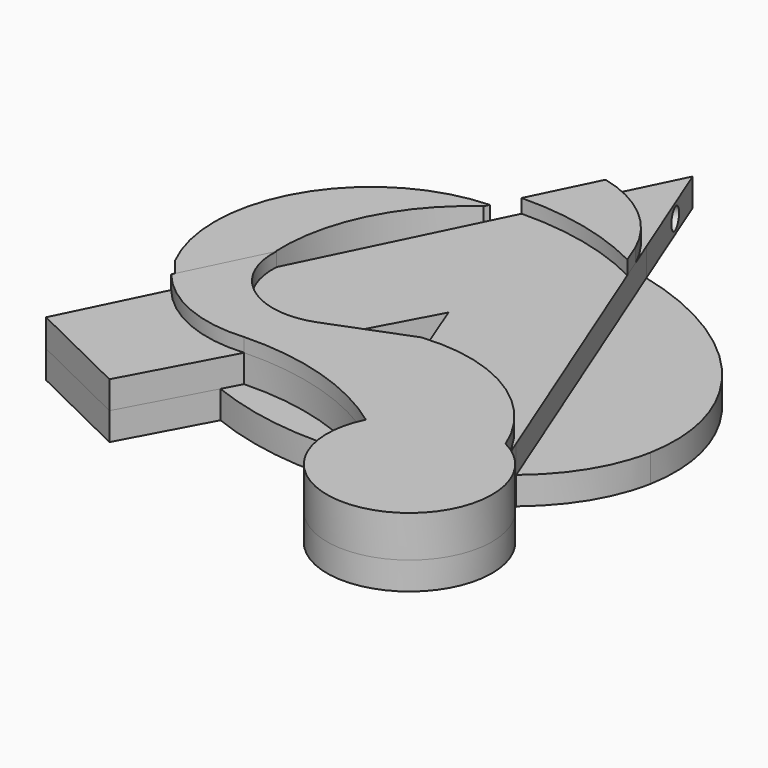
from build123d import *

# Parameters (mm, degrees)
F1_DEPTH  = 5.08
F3_DEPTH  = 5.08
F5_DEPTH  = 2.54
F7_DEPTH  = 10.16
F8_DEPTH  = 5.08
F9_DEPTH  = 5.08
F11_DEPTH = 7.62
F12_DEPTH = 2.54
F13_R     = 1.905


with BuildPart() as f1:
    # F0 (on Top) → F1 (new body)
    with BuildSketch(Plane.XY):
        with BuildLine():
            add(Edge.make_bspline(
                [(-53.1635676672, -40.7425994368), (-41.8989411061, 18.6911877843), (-113.0400156659, 1.3903249669), (-184.1810902258, -15.9105378505), (-124.304642227, -58.0434622542), (-64.4281942283, -100.1763866579), (-53.1635676672, -40.7425994368)],
                knots=[0, 0, 0, 2.0943951024, 2.0943951024, 4.1887902048, 4.1887902048, 6.2831853072, 6.2831853072, 6.2831853072], degree=2, weights=[1, 0.5, 1, 0.5, 1, 0.5, 1]))
        make_face()
    extrude(amount=F1_DEPTH)

    # F2 (on face) → F3 (join)
    with BuildSketch(Plane.XY.offset(5.08)):
        with BuildLine():
            Line((-131.9579197109, -51.2809136758), (-140.9604847431, -69.6664303541))
            Line((-140.9604847431, -69.6664303541), (-121.8411935672, -79.0282919321))
            Line((-121.8411935672, -79.0282919321), (-113.6531802251, -63.7810597846))
            add(Edge.make_bspline(
                [(-131.9579197109, -51.2809136758), (-128.6186368439, -55.0078578531), (-124.304642227, -58.0434622542), (-119.420845427, -61.4800161624), (-113.6531802251, -63.7810597846)],
                knots=[3.9072776048, 3.9072776048, 3.9072776048, 4.1887902048, 4.1887902048, 4.50468154, 4.50468154, 4.50468154], degree=2, weights=[0.8836543185, 0.9327938173, 1, 0.9245864988, 0.8719217822]))
        make_face()
        with BuildLine():
            Line((-105.5654466698, 2.6191971859), (-131.9579197109, -51.2809136758))
            add(Edge.make_bspline(
                [(-131.9579197109, -51.2809136758), (-128.6186368439, -55.0078578531), (-124.304642227, -58.0434622542), (-119.420845427, -61.4800161624), (-113.6531802251, -63.7810597846)],
                knots=[3.9072776048, 3.9072776048, 3.9072776048, 4.1887902048, 4.1887902048, 4.50468154, 4.50468154, 4.50468154], degree=2, weights=[0.8836543185, 0.9327938173, 1, 0.9245864988, 0.8719217822]))
            Line((-113.6531802251, -63.7810597846), (-96.8360751867, -32.4652455747))
            Line((-96.8360751867, -32.4652455747), (-83.3206423237, -66.8956124574))
            add(Edge.make_bspline(
                [(-83.3206423237, -66.8956124574), (-71.8467350955, -64.7720622624), (-63.8384492188, -58.1680738766)],
                knots=[5.1773121683, 5.1773121683, 5.1773121683, 5.6685915269, 5.6685915269, 5.6685915269], degree=2, weights=[0.7507848699, 0.7442133059, 0.7926641772]))
            Line((-63.8384492188, -58.1680738766), (-87.4642972057, 1.227759617))
            add(Edge.make_bspline(
                [(-87.4642972057, 1.227759617), (-96.5007837018, 3.4317958299), (-105.5654466698, 2.6191971859)],
                knots=[1.4695457005, 1.4695457005, 1.4695457005, 1.8905356916, 1.8905356916, 1.8905356916], degree=2, weights=[0.7906652984, 0.8311998282, 0.9121385395]))
        make_face()
        with BuildLine():
            add(Edge.make_bspline(
                [(-83.3206423237, -66.8956124574), (-71.8467350955, -64.7720622624), (-63.8384492188, -58.1680738766)],
                knots=[5.1773121683, 5.1773121683, 5.1773121683, 5.6685915269, 5.6685915269, 5.6685915269], degree=2, weights=[0.7507848699, 0.7442133059, 0.7926641772]))
            Line((-83.3206423237, -66.8956124574), (-82.2329744697, -69.6664303541))
            ThreePointArc((-82.2329744697, -69.6664303541), (-63.9982257769, -90.9472868448), (-61.9164295495, -63.0000680685))
            Line((-61.9164295495, -63.0000680685), (-63.8384492188, -58.1680738766))
        make_face()
        with BuildLine():
            Line((-95.8831459284, 22.3929062486), (-105.5654466698, 2.6191971859))
            add(Edge.make_bspline(
                [(-87.4642972057, 1.227759617), (-96.5007837018, 3.4317958299), (-105.5654466698, 2.6191971859)],
                knots=[1.4695457005, 1.4695457005, 1.4695457005, 1.8905356916, 1.8905356916, 1.8905356916], degree=2, weights=[0.7906652984, 0.8311998282, 0.9121385395]))
            Line((-87.4642972057, 1.227759617), (-95.8831459284, 22.3929062486))
        make_face()
    extrude(amount=F3_DEPTH)

    # F4 (on face) → F5 (join)
    with BuildSketch(Plane.XY.offset(10.16)):
        with BuildLine():
            ThreePointArc((-82.2329744697, -69.6664303541), (-63.9982257769, -90.9472868448), (-61.9164295495, -63.0000680685))
            ThreePointArc((-61.9164295495, -63.0000680685), (-73.905031166, -48.8285086128), (-92.013752266, -44.7500424488))
            Line((-92.013752266, -44.7500424488), (-82.2329744697, -69.6664303541))
        make_face()
        with BuildLine():
            Line((-82.2329744697, -69.6664303541), (-92.013752266, -44.7500424488))
            Line((-92.013752266, -44.7500424488), (-106.4470403828, -50.3622141534))
            Line((-106.4470403828, -50.3622141534), (-111.9039820196, -60.5238067737))
            ThreePointArc((-111.9039820196, -60.5238067737), (-96.3007764713, -62.6036581083), (-82.2329744697, -69.6664303541))
        make_face()
        with BuildLine():
            Line((-111.9039820196, -60.5238067737), (-106.4470403828, -50.3622141534))
            ThreePointArc((-106.4470403828, -50.3622141534), (-119.3794542725, -48.6548728117), (-124.8804196152, -36.8268669033))
            Line((-124.8804196152, -36.8268669033), (-132.2383726809, -51.8536696336))
            ThreePointArc((-132.2383726809, -51.8536696336), (-123.1504906465, -58.7200912674), (-111.9039820196, -60.5238067737))
        make_face()
    extrude(amount=F5_DEPTH)

    # F7 (add): a face of the model
    f7_faces = [f1.faces().sort_by_distance(p)[0] for p in [
        (-96.5809599227, -56.2228804189, 10.16),
    ]]
    extrude(f7_faces, amount=F7_DEPTH)

    # F8 (add): a face of the model
    f8_faces = [f1.faces().sort_by_distance(p)[0] for p in [
        (-127.5392459391, -66.1235419856, 5.08),
    ]]
    extrude(f8_faces, amount=F8_DEPTH)

    # F9 (add): a face of the model
    f9_faces = [f1.faces().sort_by_distance(p)[0] for p in [
        (-68.6388215129, -76.4740185579, 5.08),
    ]]
    extrude(f9_faces, amount=F9_DEPTH)

    # F6 (on face) → F11 (join)
    with BuildSketch(Plane.XY.offset(5.08)):
        with BuildLine():
            Line((-110.4541125519, -7.3646960477), (-110.0173115332, -6.472637797))
            ThreePointArc((-110.0173115332, -6.472637797), (-133.6523206327, -20.6370610227), (-134.4729876641, -48.1792295299))
            add(Edge.make_bspline(
                [(-134.4729876641, -48.1792295299), (-133.3080685152, -49.7740244947), (-131.9579197109, -51.2809136758)],
                knots=[3.801700486, 3.801700486, 3.801700486, 3.9072776048, 3.9072776048, 3.9072776048], degree=2, weights=[0.8493373441, 0.8652252795, 0.8836543185]))
            Line((-131.9579197109, -51.2809136758), (-125.0028994796, -37.0770017905))
            ThreePointArc((-125.0028994796, -37.0770017905), (-121.5386762873, -20.355178987), (-110.4541125519, -7.3646960477))
        make_face()
    extrude(amount=F11_DEPTH)

    # F10 (on face) → F12 (join)
    with BuildSketch(Plane.XY.offset(10.16)):
        with BuildLine():
            ThreePointArc((-107.8121787601, -1.9691984736), (-95.5792010439, -3.2282254929), (-84.0211259134, -7.428438835))
            Line((-84.0211259134, -7.428438835), (-85.4962270154, -3.7200064649))
            ThreePointArc((-85.4962270154, -3.7200064649), (-92.128084348, 5.0538321922), (-101.9519128194, 9.9989480276))
            Line((-101.9519128194, 9.9989480276), (-107.8121787601, -1.9691984736))
        make_face()
    extrude(amount=F12_DEPTH)

    # F13 (on face) → F14 (revolve, cut)
    with BuildSketch(Plane(origin=(-75.09444818, -29.8702773075, 0), x_dir=(-0.3696032606, 0.9291896629, 0), z_dir=(0.9291896629, 0.3696032606, 0))):
        with Locations((47.6521402597, 7.62)):
            Circle(F13_R)
    revolve(axis=Axis((-95.8831459284, 22.3929062486, 7.62), (0, 0, -1)), mode=Mode.SUBTRACT)


solid = f1.part
